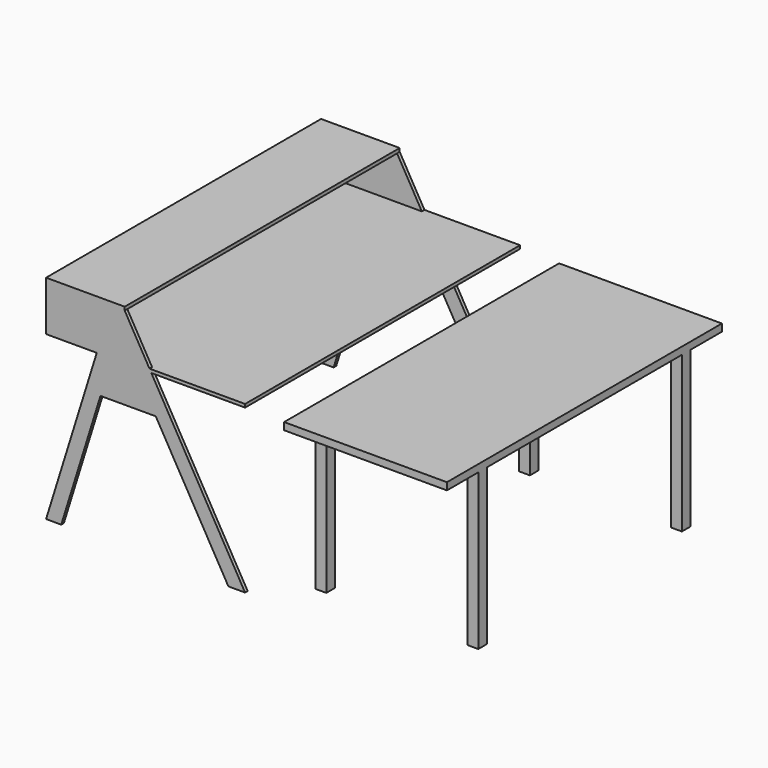
from build123d import *

# Parameters (mm, degrees)
F0_W     = 1100
F0_H     = 1900
F1_DEPTH = 1500
F0_W_2   = 900
F2_DEPTH = 900
F3_W     = 780
F3_H     = 860
F4_DEPTH = 1900
F5_START = -18
F5_DEPTH = 1864
F8_W     = 216.5617644787
F8_H     = 860
F8_W_2   = 1346.8764710426
F9_DEPTH = 900


# Not quite as in the source:
# - a feature of the source that left no trace in its solid (it failed there, or was rolled back) is left out


with BuildPart() as f1:
    # F0 (on Top) → F1 (new body)
    with BuildSketch(Plane.XY):
        with Locations((583.3312265575, 950)):
            Rectangle(F0_W, F0_H)
    extrude(amount=F1_DEPTH)


with BuildPart() as f2:
    # F0 (on Top) → F2 (new body)
    with BuildSketch(Plane.XY):
        with Locations((1799.0458726883, 950)):
            Rectangle(F0_W_2, F0_H)
    extrude(amount=F2_DEPTH)


with BuildPart() as f4_tool:
    # F3 (on face) → F4 (new body, through all)
    with BuildSketch(Plane.XZ):
        Polygon((33.3312265575, 900), (33.3312265575, 0), (313.4037852287, 900), align=None)
        Polygon((334.0880279243, 697.2315277786), (117.1153412896, 0), (1041.0203720349, 0), (639.6110557539, 697.2315277786), align=None)
        Polygon((615.1842835989, 900), (1133.3312265575, 0), (1133.3312265575, 900), (769.4745531541, 900), align=None)
        Polygon((33.3312265575, 1500), (33.3312265575, 1174.7411898097), (467.9492661672, 1174.7411898097), (467.9492661672, 1155.7411898097), (604.8213447397, 918), (1133.3312265575, 918), (1133.3312265575, 1500), align=None)
        with Locations((1799.0458726883, 430)):
            Rectangle(F3_W, F3_H)
    extrude(amount=-F4_DEPTH)


with BuildPart() as f1_1:
    add(f1.part)

    # F4: cut by f4_tool
    add(f4_tool.part, mode=Mode.SUBTRACT)

    # F3 (on face) → F5 (cut)
    with BuildSketch(Plane.XZ.offset(F5_START)):
        Polygon((313.4037852287, 900), (33.3312265575, 0), (117.1153412896, 0), (334.0880279243, 697.2315277786), (397.1878999609, 900), align=None)
        Polygon((522.8734290762, 900), (397.1878999609, 900), (334.0880279243, 697.2315277786), (639.6110557539, 697.2315277786), align=None)
        Polygon((33.3312265575, 1155.7411898097), (33.3312265575, 918), (512.5104902171, 918), (375.6384116446, 1155.7411898097), align=None)
        Polygon((639.6110557539, 697.2315277786), (1041.0203720349, 0), (1133.3312265575, 0), (615.1842835989, 900), (522.8734290762, 900), align=None)
        Polygon((375.6384116446, 1155.7411898097), (512.5104902171, 918), (584.0514024721, 918), (447.1793238996, 1155.7411898097), align=None)
        Polygon((447.1793238996, 1155.7411898097), (584.0514024721, 918), (604.8213447397, 918), (467.9492661672, 1155.7411898097), align=None)
    extrude(amount=-F5_DEPTH, mode=Mode.SUBTRACT)


with BuildPart() as f2_1:
    add(f2.part)

    # F4: cut by f4_tool
    add(f4_tool.part, mode=Mode.SUBTRACT)

    # F8 (on face) → F9 (cut, through all)
    with BuildSketch(Plane.YZ.offset(2249.0458726883)):
        with Locations((108.2808822393, 430)):
            Rectangle(F8_W, F8_H)
        with Locations((950, 430)):
            Rectangle(F8_W_2, F8_H)
        with Locations((1791.7191177607, 430)):
            Rectangle(F8_W, F8_H)
    extrude(amount=-F9_DEPTH, mode=Mode.SUBTRACT)


solid = Compound([f1_1.part, f2_1.part])
